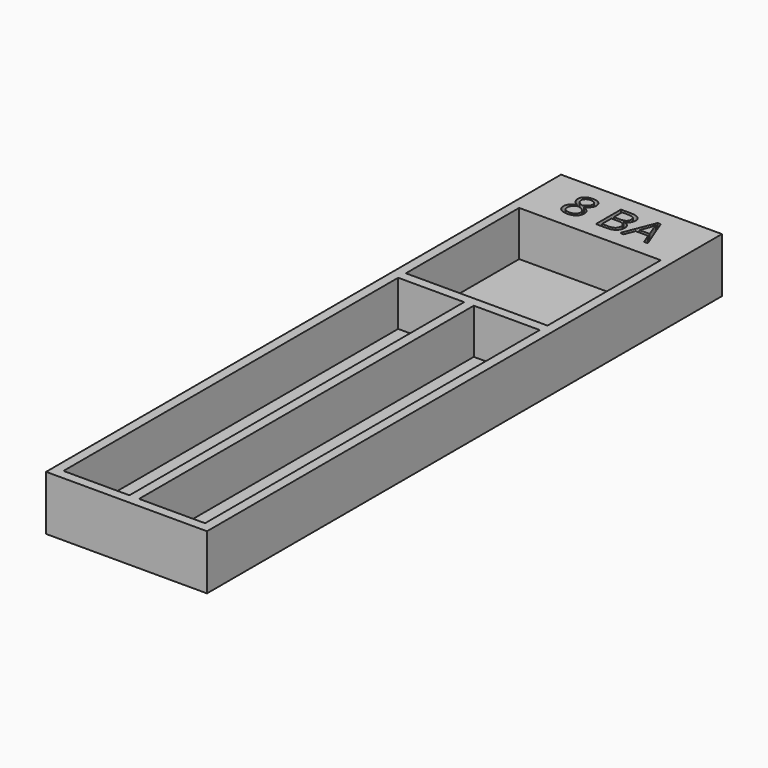
from build123d import *

# Parameters (mm, degrees)
F0_W         = 25
F0_H         = 100
F1_DEPTH     = 0.75
F2_W         = 1.5
F2_H         = 65
F3_DEPTH     = 7
F4_TEXT_SIZE = 6.8289271617
F5_DEPTH     = 1.5


# Not quite as in the source:
# - Text() gives the source's letters only with a copy of the font that has no kerning and outlines rounded to 1/6400 em; it was checked with that copy


with BuildPart() as f1:
    # F0 (on Top) → F1 (new body, symmetric)
    with BuildSketch(Plane.XY):
        with Locations((8.155064851, 32.0954295265)):
            Rectangle(F0_W, F0_H)
    extrude(amount=F1_DEPTH, both=True)

    # F2 (on face) → F3 (join)
    with BuildSketch(Plane.XY.offset(0.75)):
        Polygon((-4.344935149, -17.9045704735), (2.655064851, -17.9045704735), (4.655064851, -17.9045704735), (20.655064851, -17.9045704735), (20.655064851, 82.0954295265), (-4.344935149, 82.0954295265), align=None)
        Polygon((-2.844935149, 50.0954295265), (-2.844935149, 72.0954295265), (19.155064851, 72.0954295265), (19.155064851, 50.0954295265), (19.155064851, 48.5954295265), (19.155064851, -16.4045704735), (8.905064851, -16.4045704735), (7.405064851, -16.4045704735), (-2.844935149, -16.4045704735), (-2.844935149, 48.5954295265), align=None, mode=Mode.SUBTRACT)
        Polygon((19.155064851, 50.0954295265), (-2.844935149, 50.0954295265), (-2.844935149, 48.5954295265), (7.405064851, 48.5954295265), (8.905064851, 48.5954295265), (19.155064851, 48.5954295265), align=None)
        with Locations((8.155064851, 16.0954295265)):
            Rectangle(F2_W, F2_H)
    extrude(amount=F3_DEPTH)

    # F4 (on face) → F5 (cut)
    with BuildSketch(Plane.XY.offset(7.75)):
        with Locations((0.7211374237, 74.5954295265)):
            Text('8 BA', F4_TEXT_SIZE, font='Open Sans', text_align=(TextAlign.LEFT, TextAlign.BOTTOM))
    extrude(amount=-F5_DEPTH, mode=Mode.SUBTRACT)


solid = f1.part
